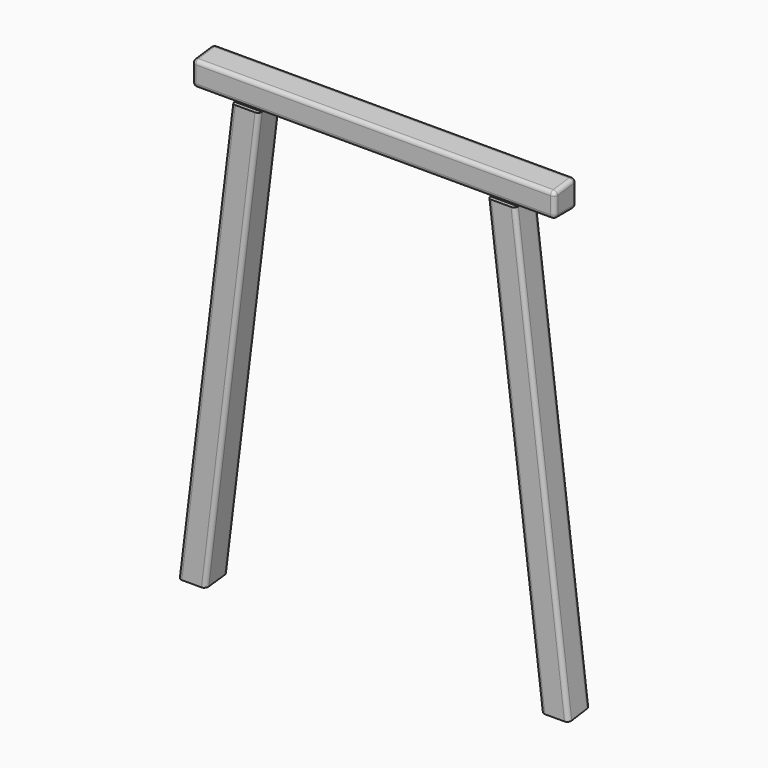
from build123d import *

# Parameters (mm, degrees)
F0_W     = 45.72
F0_H     = 3.47472
F1_DEPTH = 3.47472
F3_DEPTH = 3.47472
F5_DEPTH = 38.1
F6_W     = 45.72
F6_H     = 0.254
F7_DEPTH = 0.508
F8_R     = 0.50799


# Not quite as in the source:
# - a fillet or chamfer is up to 0.001 mm smaller than in the source, because OpenCascade refuses the exact size


with BuildPart() as f1:
    # F0 (on Front) → F1 (new body)
    with BuildSketch(Plane.XZ):
        with Locations((0, -4.3103059118)):
            Rectangle(F0_W, F0_H)
    extrude(amount=F1_DEPTH)

    # F2 (on face) → F3 (join)
    with BuildSketch(Plane.XZ.offset(3.47472)):
        Polygon((-13.929602997, -2.5729459118), (-17.4304175377, -2.5729459118), (-24.6292689013, -61.2028853004), (-21.1804489373, -61.6263471453), align=None)
        Polygon((21.1804489373, -61.6263471453), (24.6292689013, -61.2028853004), (17.4304175377, -2.5729459118), (13.929602997, -2.5729459118), align=None)
    extrude(amount=-F3_DEPTH)

    # F4 (on Right) → F5 (cut, symmetric)
    with BuildSketch(Plane.YZ):
        Polygon((-3.47472, -2.9995878813), (0, -2.5729459118), (-3.47472, -2.5729459118), align=None)
        Polygon((0, -60.7762433309), (-3.47472, -61.2028853004), (-3.47472, -61.962287873), (0, -61.962287873), align=None)
    extrude(amount=F5_DEPTH, both=True, mode=Mode.SUBTRACT)

    # F6 (on face) → F7 (cut)
    with BuildSketch(Plane.XZ.offset(3.47472)):
        with Locations((0, -6.1746659118)):
            Rectangle(F6_W, F6_H)
    extrude(amount=-F7_DEPTH, mode=Mode.SUBTRACT)

    # F8 (radius 0.508 in the source; OpenCascade refuses exactly that, so slightly less here)
    f8_edges = [f1.edges().sort_by_distance(p)[0] for p in [
        (0, -3.47472, -2.999588),
        (22.86, 0, -4.310306),
        (22.86, -1.73736, -6.047666),
        (22.86, -3.47472, -4.523627),
        (22.86, -1.73736, -2.786267),
        (21.258758, -3.47472, -33.752276),
        (-17.757943, -3.47472, -33.752276),
        (-21.258758, -3.47472, -33.752276),
        (-22.86, 0, -4.310306),
        (-22.86, -1.73736, -2.786267),
        (-22.86, -3.47472, -4.523627),
        (-22.86, -1.73736, -6.047666),
        (17.757943, -3.47472, -33.752276),
        (20.35853, 0, -6.047666),
        (17.716157, 0, -33.411955),
        (0, 0, -6.047666),
        (-20.35853, 0, -6.047666),
        (-21.216972, 0, -33.411955),
        (-17.716157, 0, -33.411955),
        (21.216972, 0, -33.411955),
        (0, -3.47472, -6.047666),
        (0, 0, -2.572946),
    ]]
    fillet(f8_edges, radius=F8_R)


solid = f1.part
